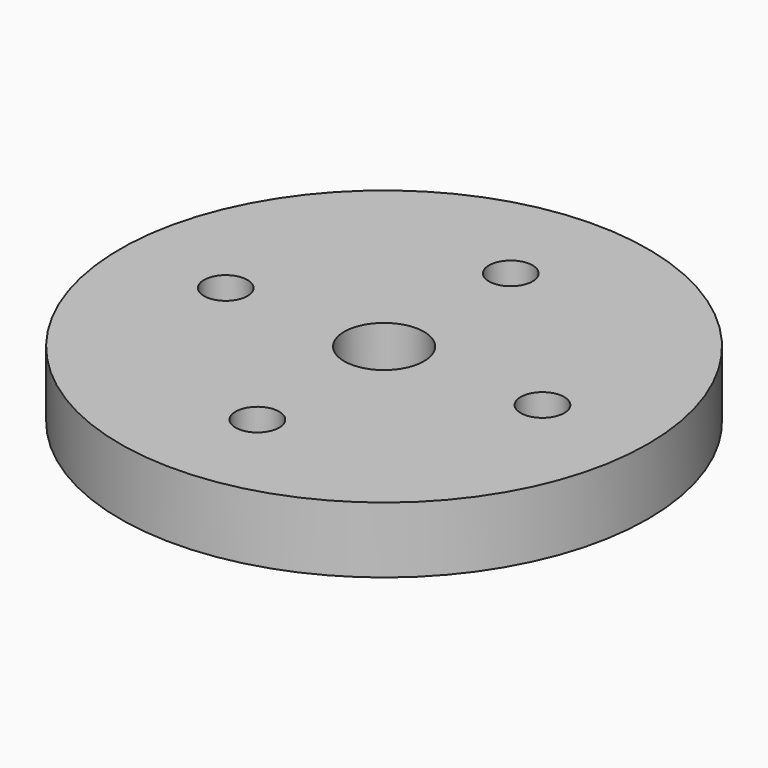
from build123d import *

# Parameters (mm, degrees)
F0_R            = 20
F1_DEPTH        = 5
F3_D            = 3.3
F3_COPIES_COUNT = 4
F5_D            = 6.05


# Not quite as in the source:
# - a pattern or mirror of a feature is missing from the dataset's text; its kind, count and spacing are read off the source's solid


with BuildPart() as f1:
    # F0 (on Top) → F1 (new body)
    with BuildSketch(Plane.XY):
        Circle(F0_R)
    extrude(amount=F1_DEPTH)

    # F3 (through all)
    with Locations(Plane.XY.offset(5)):
        with Locations((0, 12)):
            f3 = Hole(F3_D / 2)

    # F3_copies: F3 ×4 about axis
    f3_copies_axis = Axis((0, 0, 0), (0, 0, 1))
    for i in range(1, F3_COPIES_COUNT):
        add(f3.rotate(f3_copies_axis, i * 360 / F3_COPIES_COUNT), mode=Mode.SUBTRACT)

    # F5 (through all)
    with Locations(Plane.XY.offset(5)):
        with Locations((0, 0)):
            Hole(F5_D / 2)


solid = f1.part
